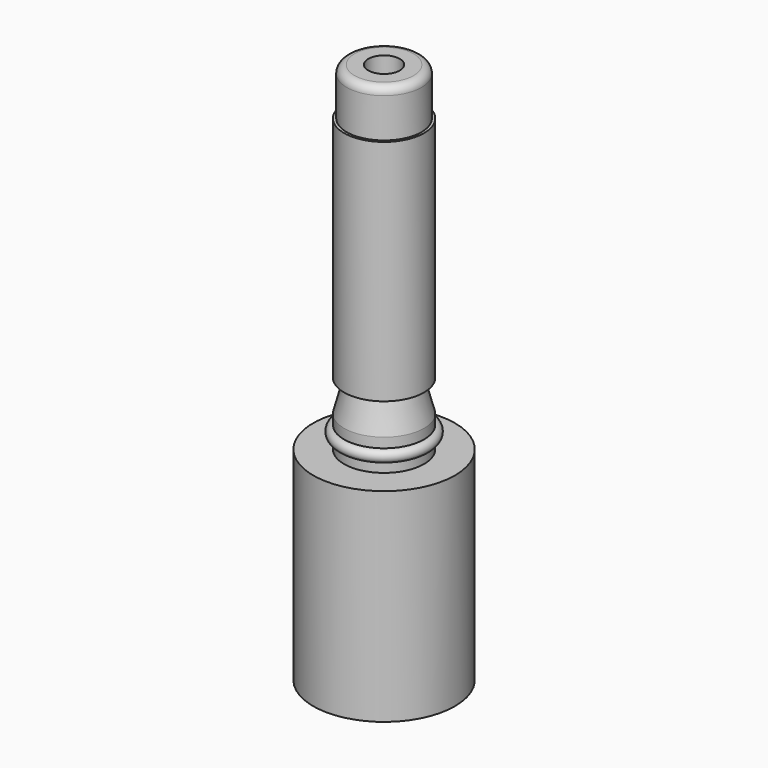
from build123d import *

# Parameters (mm, degrees)
F0_R      = 5.08
F1_DEPTH  = 37
F2_R      = 9
F3_DEPTH  = 2
F4_R      = 9
F4_R_2    = 7.75
F5_DEPTH  = 23.8
F6_R      = 4.75
F7_DEPTH  = 6
F8_R      = 1
F13_R     = 2
F14_DEPTH = 25


with BuildPart() as f1:
    # F0 (on Top) → F1 (new body)
    with BuildSketch(Plane.XY):
        Circle(F0_R)
    extrude(amount=F1_DEPTH)

    # F2 (on face) → F3 (join)
    with BuildSketch(Plane(origin=(0, 0, 0), x_dir=(1, 0, 0), z_dir=(0, 0, -1))):
        Circle(F2_R)
    extrude(amount=F3_DEPTH)

    # F4 (on face) → F5 (join)
    with BuildSketch(Plane(origin=(0, 0, -2), x_dir=(1, 0, 0), z_dir=(0, 0, -1))):
        Circle(F4_R)
        Circle(F4_R_2, mode=Mode.SUBTRACT)
    extrude(amount=F5_DEPTH)

    # F9 (on Front) → F10 (revolve, cut)
    with BuildSketch(Plane.XZ):
        Polygon((-5.08, 8), (-5.08, 4), (-4.0082032303, 8), align=None)
    revolve(axis=Axis((0, 0, 0), (0, 0, -1)), mode=Mode.SUBTRACT)

    # F9 (on Front) → F11 (revolve, cut)
    with BuildSketch(Plane.XZ):
        with BuildLine():
            Line((-5.08, 1.25), (-5.08, 2.75))
            ThreePointArc((-5.08, 2.75), (-5.83, 2), (-5.08, 1.25))
        make_face()
        with BuildLine():
            ThreePointArc((-4.33, 2), (-4.5496699141, 2.5303300859), (-5.08, 2.75))
            Line((-5.08, 2.75), (-5.08, 1.25))
            ThreePointArc((-5.08, 1.25), (-4.5496699141, 1.4696699141), (-4.33, 2))
        make_face()
    revolve(axis=Axis((0, 0, 0), (0, 0, -1)), mode=Mode.SUBTRACT)


with BuildPart() as f7:
    # F6 (on face) → F7 (new body)
    with BuildSketch(Plane.XY.offset(37)):
        Circle(F6_R)
    extrude(amount=F7_DEPTH)

    # F8
    f8_edges = [f7.edges().sort_by_distance(p)[0] for p in [
        (-4.75, 0, 43),
    ]]
    fillet(f8_edges, radius=F8_R)


with BuildPart() as f12:
    # F9 (on Front) → F12 (revolve)
    with BuildSketch(Plane.XZ):
        with BuildLine():
            ThreePointArc((-4.33, 2), (-4.5496699141, 2.5303300859), (-5.08, 2.75))
            Line((-5.08, 2.75), (-5.08, 1.25))
            ThreePointArc((-5.08, 1.25), (-4.5496699141, 1.4696699141), (-4.33, 2))
        make_face()
        with BuildLine():
            Line((-5.08, 1.25), (-5.08, 2.75))
            ThreePointArc((-5.08, 2.75), (-5.83, 2), (-5.08, 1.25))
        make_face()
    revolve(axis=Axis((0, 0, 0), (0, 0, -1)))


with BuildPart() as f14_tool:
    # F13 (on face) → F14 (new body)
    with BuildSketch(Plane.XY.offset(43)):
        Circle(F13_R)
    extrude(amount=-F14_DEPTH)


with BuildPart() as f1_1:
    add(f1.part)

    # F14: cut by f14_tool
    add(f14_tool.part, mode=Mode.SUBTRACT)


with BuildPart() as f7_1:
    add(f7.part)

    # F14: cut by f14_tool
    add(f14_tool.part, mode=Mode.SUBTRACT)


solid = Compound([f12.part, f1_1.part, f7_1.part])
